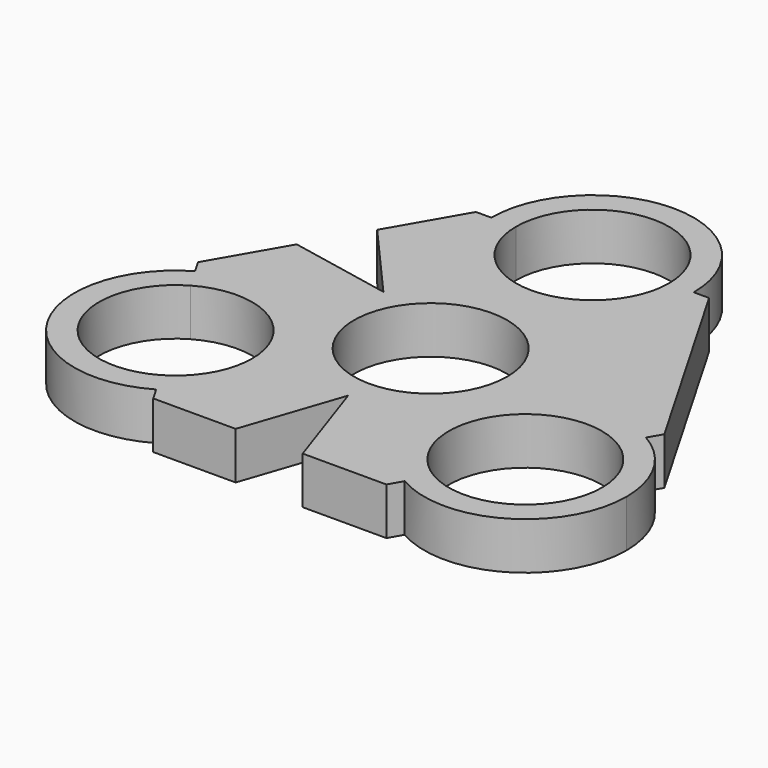
from build123d import *

# Parameters (mm, degrees)
F0_R     = 11.35
F1_DEPTH = 7
F3_DEPTH = 50.7


# Not quite as in the source:
# - a feature names something its author has since deleted; it is built from what else it names


with BuildPart() as f1:
    # F0 (on Top) → F1 (new body)
    with BuildSketch(Plane.XY):
        with BuildLine():
            Line((-31.5669890957, -5.0726587053), (-33.3938997814, -1.9127698865))
            ThreePointArc((-33.3938997814, -1.9127698865), (-38.8718921093, -22.4064664798), (-18.378195516, -27.8844588077))
            Line((-18.378195516, -27.8844588077), (-20.2051062016, -24.7245699889))
            ThreePointArc((-20.2051062016, -24.7245699889), (-35.7120032905, -20.5795557942), (-31.5669890957, -5.0726587053))
        make_face()
        with BuildLine():
            ThreePointArc((-10.8860476487, -14.8986143471), (-18.3899747432, -1.9059667726), (-33.3938997814, -1.9127698865))
            Line((-33.3938997814, -1.9127698865), (-31.5669890957, -5.0726587053))
            ThreePointArc((-31.5669890957, -5.0726587053), (-20.2140191502, -5.0675110157), (-14.5360476487, -14.8986143471))
            ThreePointArc((-14.5360476487, -14.8986143471), (-16.0549443173, -20.5706428456), (-20.2051062016, -24.7245699889))
            Line((-20.2051062016, -24.7245699889), (-18.378195516, -27.8844588077))
            ThreePointArc((-18.378195516, -27.8844588077), (-12.8934000742, -22.3946872526), (-10.8860476487, -14.8986143471))
        make_face()
        with BuildLine():
            ThreePointArc((-11.3499979258, 29.9931382104), (-0.0068617896, 41.3499979258), (11.3499979258, 30.0068617896))
            Line((11.3499979258, 30.0068617896), (14.9999972588, 30.0090684445))
            ThreePointArc((14.9999972588, 30.0090684445), (-0.0090684445, 44.9999972588), (-14.9999972588, 29.9909315555))
            Line((-14.9999972588, 29.9909315555), (-11.3499979258, 29.9931382104))
        make_face()
        with BuildLine():
            ThreePointArc((11.3499979258, 30.0068617896), (11.3499994815, 30.003430895), (11.35, 30))
            ThreePointArc((11.35, 30), (0.003430895, 18.6500005185), (-11.3499979258, 29.9931382104))
            Line((-11.3499979258, 29.9931382104), (-14.9999972588, 29.9909315555))
            ThreePointArc((-14.9999972588, 29.9909315555), (0.0045342224, 15.0000006853), (15, 30))
            ThreePointArc((15, 30), (14.9999993147, 30.0045342224), (14.9999972588, 30.0090684445))
            Line((14.9999972588, 30.0090684445), (11.3499979258, 30.0068617896))
        make_face()
        with BuildLine():
            Line((31.6093732737, -5.0344646094), (33.4324619211, -1.8723691359))
            ThreePointArc((33.4324619211, -1.8723691359), (12.9454038899, -7.3751369148), (18.4481716689, -27.8621949459))
            Line((18.4481716689, -27.8621949459), (20.2712603162, -24.7000994724))
            ThreePointArc((20.2712603162, -24.7000994724), (16.1074993635, -9.1982255621), (31.6093732737, -5.0344646094))
        make_face()
        with BuildLine():
            ThreePointArc((40.940316795, -14.8672820409), (38.928430147, -7.3633556317), (33.4324619211, -1.8723691359))
            Line((33.4324619211, -1.8723691359), (31.6093732737, -5.0344646094))
            ThreePointArc((31.6093732737, -5.0344646094), (35.7679892314, -9.189311058), (37.290316795, -14.8672820409))
            ThreePointArc((37.290316795, -14.8672820409), (31.6182877779, -24.6949544773), (20.2712603162, -24.7000994724))
            Line((20.2712603162, -24.7000994724), (18.4481716689, -27.8621949459))
            ThreePointArc((18.4481716689, -27.8621949459), (33.4442432041, -27.855395393), (40.940316795, -14.8672820409))
        make_face()
        with BuildLine():
            Line((17.2754548146, 30.0104441021), (14.9999972588, 30.0090684445))
            ThreePointArc((14.9999972588, 30.0090684445), (14.9999993147, 30.0045342224), (15, 30))
            ThreePointArc((15, 30), (0.0045342224, 15.0000006853), (-14.9999972588, 29.9909315555))
            Line((-14.9999972588, 29.9909315555), (-17.2754548146, 29.9895558979))
            Line((-17.2754548146, 29.9895558979), (-34.5328199137, 0.0571463332))
            Line((-34.5328199137, 0.0571463332), (-33.3938997814, -1.9127698865))
            ThreePointArc((-33.3938997814, -1.9127698865), (-18.3899747432, -1.9059667726), (-10.8860476487, -14.8986143471))
            ThreePointArc((-10.8860476487, -14.8986143471), (-12.8934000742, -22.3946872526), (-18.378195516, -27.8844588077))
            Line((-18.378195516, -27.8844588077), (-17.2392753837, -29.8543750274))
            Line((-17.2392753837, -29.8543750274), (17.3116342454, -29.8334868233))
            Line((17.3116342454, -29.8334868233), (18.4481716689, -27.8621949459))
            ThreePointArc((18.4481716689, -27.8621949459), (12.9454038899, -7.3751369148), (33.4324619211, -1.8723691359))
            Line((33.4324619211, -1.8723691359), (34.5689993445, 0.0989227415))
            Line((34.5689993445, 0.0989227415), (17.2754548146, 30.0104441021))
        make_face()
        Circle(F0_R, mode=Mode.SUBTRACT)
    extrude(amount=F1_DEPTH)

    # F2 (on face) → F3 (cut)
    with BuildSketch(Plane.XY.offset(7)):
        Polygon((-13.1224627256, 7.654147332), (-23.4067556554, 19.3549887506), (-28.4015190728, 10.6917134805), align=None)
        Polygon((-0.067454671, -15.1914597466), (-5.0242557701, -29.8469902776), (4.9070631834, -29.8409861689), align=None)
    extrude(amount=-F3_DEPTH, mode=Mode.SUBTRACT)


solid = f1.part
